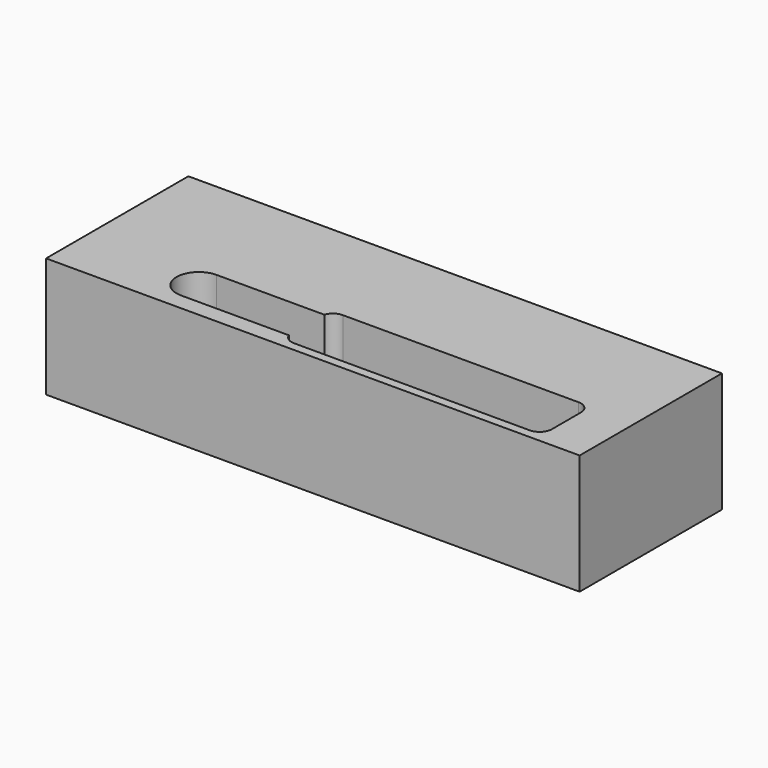
from build123d import *

# Parameters (mm, degrees)
F0_W     = 152.4
F0_H     = 50.8
F1_DEPTH = 31.7246
F2_DEPTH = 2.54
F3_DEPTH = 15.24


# Not quite as in the source:
# - a feature names something its author has since deleted; it is built from what else it names


with BuildPart() as f1:
    # F0 (on Top) → F1 (new body)
    with BuildSketch(Plane.XY):
        with Locations((76.2, 25.4)):
            Rectangle(F0_W, F0_H)
        with BuildLine():
            Line((139.6399507581, 16.4298143223), (139.6399507581, 6.0491856777))
            ThreePointArc((139.6399507581, 6.0491856777), (138.6121340696, 3.5678166885), (136.1307650805, 2.54))
            Line((136.1307650805, 2.54), (68.7885385865, 2.54))
            ThreePointArc((68.7885385865, 2.54), (66.7857906668, 3.167626223), (65.4994352256, 4.826))
            Line((65.4994352256, 4.826), (50.0925188645, 4.826))
            Line((50.0925188645, 4.826), (34.6856025033, 4.826))
            ThreePointArc((34.6856025033, 4.826), (28.3356025033, 11.176), (34.6856025033, 17.526))
            Line((34.6856025033, 17.526), (50.0925188645, 17.526))
            Line((50.0925188645, 17.526), (65.4549577669, 17.526))
            ThreePointArc((65.4549577669, 17.526), (66.7309106998, 19.2724454275), (68.7885385865, 19.939))
            Line((68.7885385865, 19.939), (136.1307650805, 19.939))
            ThreePointArc((136.1307650805, 19.939), (138.6121340696, 18.9111833115), (139.6399507581, 16.4298143223))
        make_face(mode=Mode.SUBTRACT)
    extrude(amount=F1_DEPTH)

    # F0 (on Top) → F2 (join)
    with BuildSketch(Plane.XY):
        with Locations((76.2, 25.4)):
            Rectangle(F0_W, F0_H)
        with BuildLine():
            Line((139.6399507581, 16.4298143223), (139.6399507581, 6.0491856777))
            ThreePointArc((139.6399507581, 6.0491856777), (138.6121340696, 3.5678166885), (136.1307650805, 2.54))
            Line((136.1307650805, 2.54), (68.7885385865, 2.54))
            ThreePointArc((68.7885385865, 2.54), (66.7857906668, 3.167626223), (65.4994352256, 4.826))
            Line((65.4994352256, 4.826), (50.0925188645, 4.826))
            Line((50.0925188645, 4.826), (34.6856025033, 4.826))
            ThreePointArc((34.6856025033, 4.826), (28.3356025033, 11.176), (34.6856025033, 17.526))
            Line((34.6856025033, 17.526), (50.0925188645, 17.526))
            Line((50.0925188645, 17.526), (65.4549577669, 17.526))
            ThreePointArc((65.4549577669, 17.526), (66.7309106998, 19.2724454275), (68.7885385865, 19.939))
            Line((68.7885385865, 19.939), (136.1307650805, 19.939))
            ThreePointArc((136.1307650805, 19.939), (138.6121340696, 18.9111833115), (139.6399507581, 16.4298143223))
        make_face(mode=Mode.SUBTRACT)
        with BuildLine():
            ThreePointArc((136.1307650805, 2.54), (138.6121340696, 3.5678166885), (139.6399507581, 6.0491856777))
            Line((139.6399507581, 6.0491856777), (139.6399507581, 16.4298143223))
            ThreePointArc((139.6399507581, 16.4298143223), (138.6121340696, 18.9111833115), (136.1307650805, 19.939))
            Line((136.1307650805, 19.939), (68.7885385865, 19.939))
            ThreePointArc((68.7885385865, 19.939), (66.7309106998, 19.2724454275), (65.4549577669, 17.526))
            Line((65.4549577669, 17.526), (50.0925188645, 17.526))
            ThreePointArc((50.0925188645, 17.526), (47.107835886, 11.176), (50.0925188645, 4.826))
            Line((50.0925188645, 4.826), (65.4994352256, 4.826))
            ThreePointArc((65.4994352256, 4.826), (66.7857906668, 3.167626223), (68.7885385865, 2.54))
            Line((68.7885385865, 2.54), (136.1307650805, 2.54))
        make_face()
        with BuildLine():
            ThreePointArc((92.2508400636, 8.0152933773), (89.0266334409, 11.2395), (92.2508400636, 14.4637066227))
            Line((92.2508400636, 14.4637066227), (110.0372854958, 14.4637066227))
            ThreePointArc((110.0372854958, 14.4637066227), (113.2614921185, 11.2395), (110.0372854958, 8.0152933773))
            Line((110.0372854958, 8.0152933773), (92.2508400636, 8.0152933773))
        make_face(mode=Mode.SUBTRACT)
        with BuildLine():
            Line((34.6856025033, 4.826), (50.0925188645, 4.826))
            ThreePointArc((50.0925188645, 4.826), (47.107835886, 11.176), (50.0925188645, 17.526))
            Line((50.0925188645, 17.526), (34.6856025033, 17.526))
            ThreePointArc((34.6856025033, 17.526), (28.3356025033, 11.176), (34.6856025033, 4.826))
        make_face()
    extrude(amount=-F2_DEPTH)

    # F0 (on Top) → F3 (join)
    with BuildSketch(Plane.XY):
        with BuildLine():
            Line((34.6856025033, 4.826), (50.0925188645, 4.826))
            ThreePointArc((50.0925188645, 4.826), (47.107835886, 11.176), (50.0925188645, 17.526))
            Line((50.0925188645, 17.526), (34.6856025033, 17.526))
            ThreePointArc((34.6856025033, 17.526), (28.3356025033, 11.176), (34.6856025033, 4.826))
        make_face()
    extrude(amount=F3_DEPTH)


solid = f1.part
